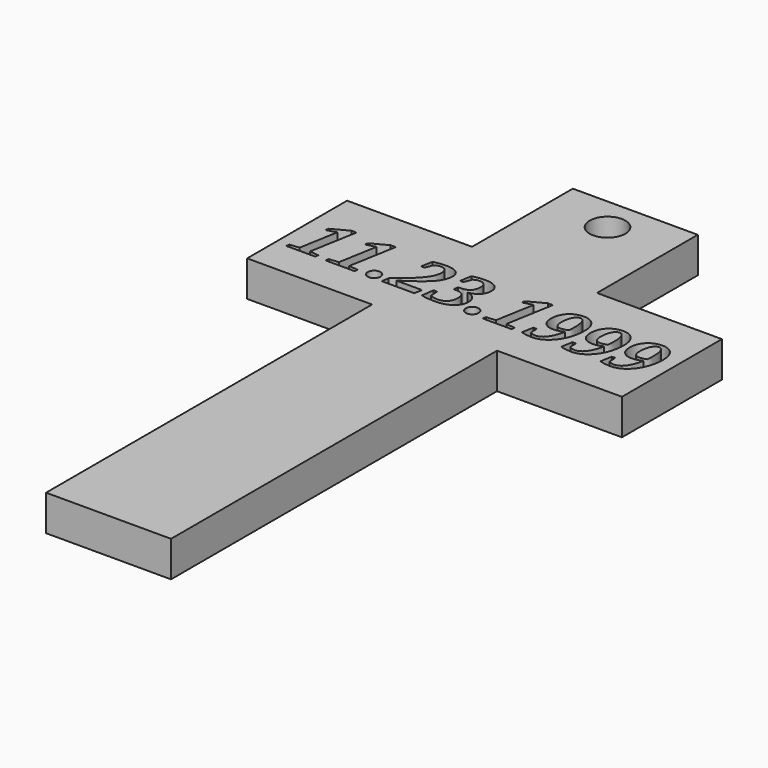
from build123d import *

# Parameters (mm, degrees)
F1_DEPTH     = 5.08
F2_TEXT_SIZE = 11.1771177118
F3_DEPTH     = 25.4
F4_R         = 2.54
F5_DEPTH     = 25.4


# Not quite as in the source:
# - Text() gives the source's letters only with a copy of the font that has no kerning and outlines rounded to 1/6400 em; it was checked with that copy


with BuildPart() as f1:
    # F0 (on Top) → F1 (new body)
    with BuildSketch(Plane.XY):
        Polygon((-0.6861395562, 41.0789623857), (-18.4661395562, 41.0789623857), (-18.4661395562, 23.149798746), (-36.2461395562, 23.149798746), (-36.2461395562, 5.369798746), (-18.4661395562, 5.369798746), (-18.4661395562, -52.6240281761), (-0.6861395562, -52.6240281761), (-0.6861395562, 5.369798746), (17.0938604438, 5.369798746), (17.0938604438, 23.149798746), (-0.6861395562, 23.149798746), align=None)
    extrude(amount=F1_DEPTH)

    # F2 (on face) → F3 (cut)
    with BuildSketch(Plane.XY.offset(5.08)):
        with Locations((-34.9853986019, 10.4233565393)):
            Text('11.23.1999', F2_TEXT_SIZE, font='Tinos', font_style=FontStyle.BOLDITALIC, text_align=(TextAlign.LEFT, TextAlign.BOTTOM))
    extrude(amount=-F3_DEPTH, mode=Mode.SUBTRACT)

    # F4 (on face) → F5 (cut)
    with BuildSketch(Plane.XY.offset(5.08)):
        with Locations((-9.6656382084, 36.2461395562)):
            Circle(F4_R)
    extrude(amount=-F5_DEPTH, mode=Mode.SUBTRACT)


solid = f1.part
